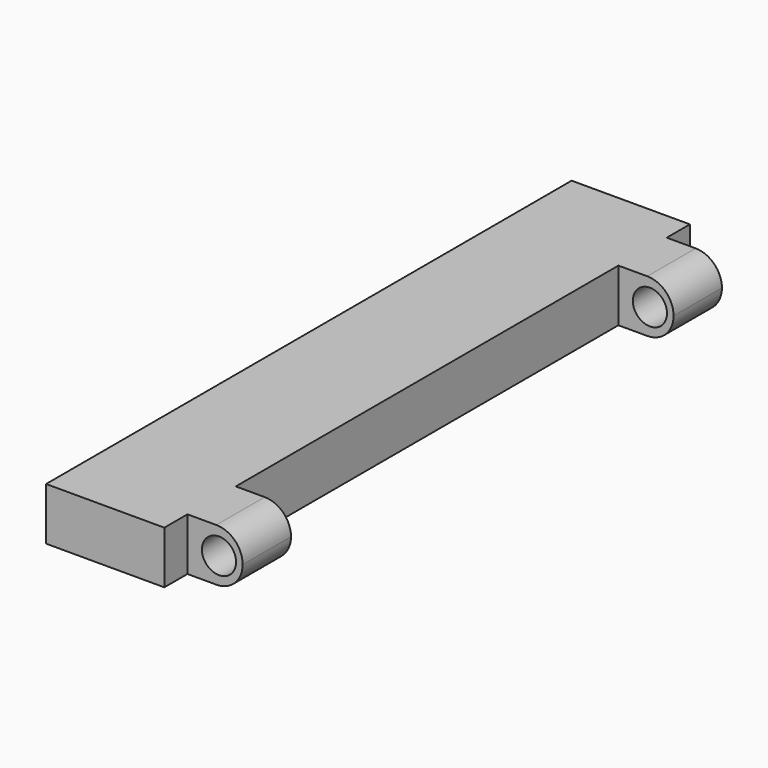
from build123d import *

# Parameters (mm, degrees)
F0_W     = 9
F0_H     = 4
F1_DEPTH = 25
F2_W     = 4.6
F2_H     = 4
F3_DEPTH = 4.2
F4_R     = 1.3
F5_DEPTH = 25
F6_R     = 1.99999


# Not quite as in the source:
# - a fillet or chamfer is up to 0.001 mm smaller than in the source, because OpenCascade refuses the exact size


with BuildPart() as f1:
    # F0 (on Front) → F1 (new body)
    with BuildSketch(Plane.XZ):
        with Locations((-22.8743378759, 29.5677930117)):
            Rectangle(F0_W, F0_H)
    extrude(amount=F1_DEPTH)

    # F2 (on face) → F3 (join)
    with BuildSketch(Plane.YZ.offset(-18.3743378759)):
        with Locations((-20.5, 29.5677930117)):
            Rectangle(F2_W, F2_H)
    extrude(amount=F3_DEPTH)

    # F4 (on face) → F5 (cut)
    with BuildSketch(Plane.XZ.offset(22.8)):
        with Locations((-15.9743378759, 29.5677930117)):
            Circle(F4_R)
    extrude(amount=-F5_DEPTH, mode=Mode.SUBTRACT)

    # F6 (radius 2 in the source; OpenCascade refuses exactly that, so slightly less here)
    f6_edges = [f1.edges().sort_by_distance(p)[0] for p in [
        (-14.174338, -20.5, 31.567793),
        (-14.174338, -20.5, 27.567793),
    ]]
    fillet(f6_edges, radius=F6_R)

    # F7: F1 across face


with BuildPart() as f1_1:
    add(f1.part)
    add(f1.part.mirror(Plane(origin=(-22.8743378759, 0, 29.5677930117), x_dir=(1, 0, 0), z_dir=(0, 1, 0))))


with BuildPart() as f8_1:
    # F8: copy of F1
    add(f1_1.part)


solid = f1_1.part
